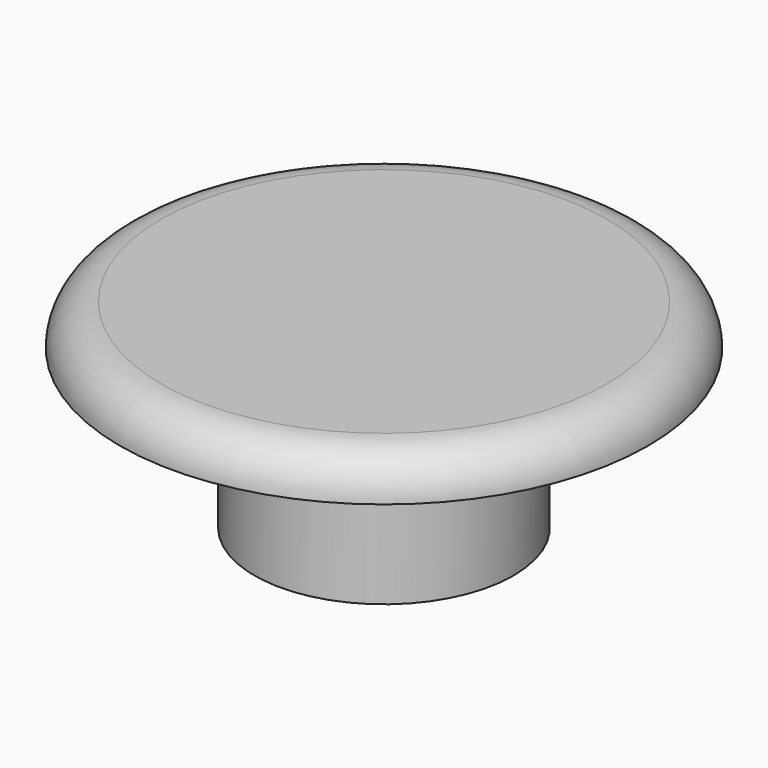
from build123d import *

# Parameters (mm, degrees)
F0_R     = 4.0005
F1_DEPTH = 3.4798
F0_R_2   = 5.0165
F2_DEPTH = 1.397
F3_R     = 8.1534
F3_R_2   = 5.0165
F4_DEPTH = 1.27
F5_R     = 1.26999


# Not quite as in the source:
# - a fillet or chamfer is up to 0.001 mm smaller than in the source, because OpenCascade refuses the exact size


with BuildPart() as f1:
    # F0 (on Top) → F1 (new body)
    with BuildSketch(Plane.XY):
        Circle(F0_R)
    extrude(amount=-F1_DEPTH)

    # F0 (on Top) → F2 (join)
    with BuildSketch(Plane.XY):
        Circle(F0_R_2)
        Circle(F0_R, mode=Mode.SUBTRACT)
        Circle(F0_R)
    extrude(amount=F2_DEPTH)

    # F3 (on face) → F4 (join)
    with BuildSketch(Plane.XY.offset(1.397)):
        Circle(F3_R)
        Circle(F3_R_2, mode=Mode.SUBTRACT)
        Circle(F3_R_2)
    extrude(amount=F4_DEPTH)

    # F5 (radius 1.27 in the source; OpenCascade refuses exactly that, so slightly less here)
    f5_edges = [f1.edges().sort_by_distance(p)[0] for p in [
        (-8.1534, 0, 2.667),
    ]]
    fillet(f5_edges, radius=F5_R)


solid = f1.part
